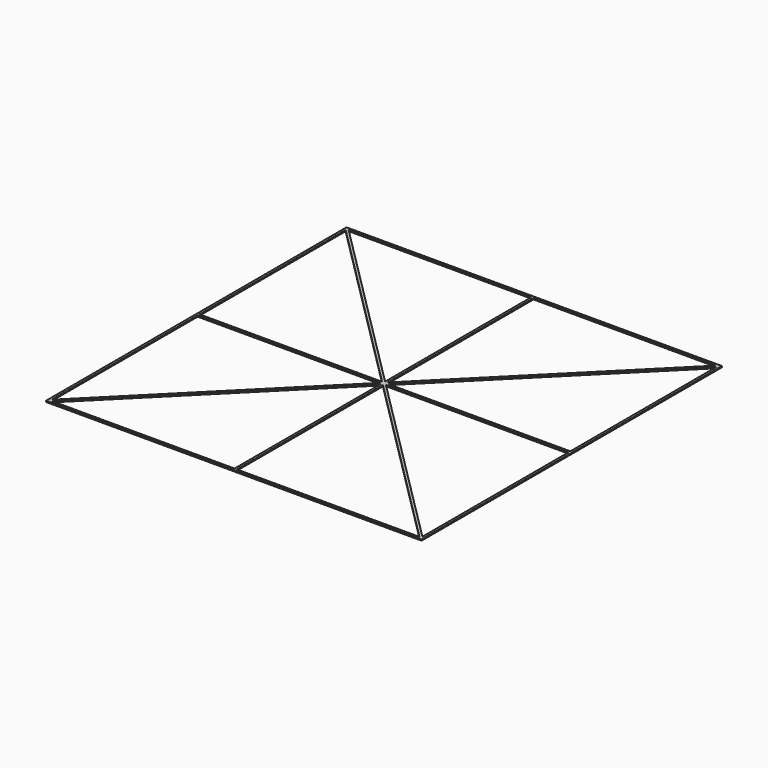
from build123d import *

# Parameters (mm, degrees)
F1_DEPTH = 0.5


# Not quite as in the source:
# - a pattern or mirror of a feature is missing from the dataset's text; its kind, count and spacing are read off the source's solid


with BuildPart() as f1:
    # F0 (on Top) → F1 (new body)
    with BuildSketch(Plane.XY):
        Polygon((160, 0), (0, 0), (0, -1), (0, -160), (160, -160), align=None)
        Polygon((1, -1.7071067812), (1, -1), (1.7071067812, -1), (79.5, -1), (80, -1), (80.5, -1), (158.2928932188, -1), (159, -1), (159, -1.7071067812), (159, -79.5), (159, -80.5), (159, -158.2928932188), (159, -159), (158.2928932188, -159), (80.5, -159), (80, -159), (79.5, -159), (1.7071067812, -159), (1, -159), (1, -158.2928932188), (1, -80.5), (1, -80), (1, -79.5), align=None, mode=Mode.SUBTRACT)
        Polygon((78.7928932188, -79.5), (1, -79.5), (1, -80), (1, -80.5), (78.7928932188, -80.5), (79.2928932188, -80), align=None)
        Polygon((159, -79.5), (81.2071067812, -79.5), (80.7071067812, -80), (81.2071067812, -80.5), (159, -80.5), align=None)
        Polygon((79.5, -78.7928932188), (1.7071067812, -1), (1.3535533906, -1.3535533906), (79.5, -79.5), align=None)
        Polygon((1.3535533906, -1.3535533906), (1, -1.7071067812), (78.7928932188, -79.5), (79.5, -79.5), align=None)
        Polygon((146.2407427602, -146.2407427602), (80.5, -80.5), (80.5, -81.2071067812), (145.8871893697, -146.5942961508), align=None)
        Polygon((81.2071067812, -80.5), (80.5, -80.5), (146.2407427602, -146.2407427602), (146.5942961508, -145.8871893697), align=None)
        Polygon((80, -1), (79.5, -1), (79.5, -78.7928932188), (80, -79.2928932188), align=None)
        Polygon((80.5, -1), (80, -1), (80, -79.2928932188), (80.5, -78.7928932188), align=None)
        Polygon((80, -80.7071067812), (79.5, -81.2071067812), (79.5, -159), (80, -159), align=None)
        Polygon((80.5, -81.2071067812), (80, -80.7071067812), (80, -159), (80.5, -159), align=None)
        Polygon((146.5942961508, -145.8871893697), (146.2407427602, -146.2407427602), (158.6464466094, -158.6464466094), (159, -158.2928932188), align=None)
        Polygon((158.6464466094, -158.6464466094), (146.2407427602, -146.2407427602), (145.8871893697, -146.5942961508), (158.2928932188, -159), align=None)
        Polygon((159, -1), (158.2928932188, -1), (149.7961722435, -9.4967209753), (150.1497256341, -9.8502743659), align=None)
        Polygon((159, -1.7071067812), (159, -1), (150.1497256341, -9.8502743659), (150.5032790247, -10.2038277565), align=None)
        Polygon((80, -79.2928932188), (79.5, -78.7928932188), (79.5, -79.5), (79.7928932188, -79.5), align=None)
        Polygon((79.5, -79.5), (78.7928932188, -79.5), (79.2928932188, -80), (79.5, -79.7928932188), align=None)
        Polygon((80.5, -78.7928932188), (80, -79.2928932188), (80.2071067812, -79.5), (80.5, -79.5), align=None)
        Polygon((79.5, -80.2071067812), (79.2928932188, -80), (78.7928932188, -80.5), (79.5, -80.5), align=None)
        Polygon((80, -80), (79.6464466094, -79.6464466094), (79.5, -79.7928932188), (79.5, -80.2071067812), (79.6464466094, -80.3535533906), align=None)
        Polygon((80.3535533906, -79.6464466094), (80, -80), (80.3535533906, -80.3535533906), (80.5, -80.2071067812), (80.5, -79.7928932188), align=None)
        Polygon((81.2071067812, -79.5), (80.5, -79.5), (80.5, -79.7928932188), (80.7071067812, -80), align=None)
        Polygon((79.7928932188, -80.5), (79.5, -80.5), (79.5, -81.2071067812), (80, -80.7071067812), align=None)
        Polygon((80.5, -80.5), (80.2071067812, -80.5), (80, -80.7071067812), (80.5, -81.2071067812), align=None)
        Polygon((80.7071067812, -80), (80.5, -80.2071067812), (80.5, -80.5), (81.2071067812, -80.5), align=None)
        Polygon((1.7071067812, -1), (1, -1), (1.3535533906, -1.3535533906), align=None)
        Polygon((1.3535533906, -1.3535533906), (1, -1), (1, -1.7071067812), align=None)
        Polygon((1.3535533906, -158.6464466094), (1, -158.2928932188), (1, -159), align=None)
        Polygon((1.3535533906, -158.6464466094), (1, -159), (1.7071067812, -159), align=None)
        Polygon((159, -158.2928932188), (158.6464466094, -158.6464466094), (159, -159), align=None)
        Polygon((159, -159), (158.6464466094, -158.6464466094), (158.2928932188, -159), align=None)
        Polygon((80, -79.5), (79.7928932188, -79.5), (79.6464466094, -79.6464466094), (80, -80), align=None)
        Polygon((80.2071067812, -79.5), (80, -79.5), (80, -80), (80.3535533906, -79.6464466094), align=None)
        Polygon((80.3535533906, -80.3535533906), (80, -80), (80, -80.5), (80.2071067812, -80.5), align=None)
        Polygon((80, -80.5), (80, -80), (79.6464466094, -80.3535533906), (79.7928932188, -80.5), align=None)
        Polygon((79.5, -79.7928932188), (79.2928932188, -80), (79.5, -80.2071067812), align=None)
        Polygon((80.7071067812, -80), (80.5, -79.7928932188), (80.5, -80.2071067812), align=None)
        Polygon((79.7928932188, -79.5), (79.5, -79.5), (79.6464466094, -79.6464466094), align=None)
        Polygon((79.6464466094, -79.6464466094), (79.5, -79.5), (79.5, -79.7928932188), align=None)
        Polygon((80.2071067812, -79.5), (80, -79.2928932188), (80, -79.5), align=None)
        Polygon((80, -79.5), (80, -79.2928932188), (79.7928932188, -79.5), align=None)
        Polygon((80.5, -79.5), (80.2071067812, -79.5), (80.3535533906, -79.6464466094), align=None)
        Polygon((79.6464466094, -80.3535533906), (79.5, -80.2071067812), (79.5, -80.5), align=None)
        Polygon((80.5, -79.7928932188), (80.5, -79.5), (80.3535533906, -79.6464466094), align=None)
        Polygon((79.6464466094, -80.3535533906), (79.5, -80.5), (79.7928932188, -80.5), align=None)
        Polygon((80, -80.7071067812), (80, -80.5), (79.7928932188, -80.5), align=None)
        Polygon((80.2071067812, -80.5), (80, -80.5), (80, -80.7071067812), align=None)
        Polygon((80.5, -80.5), (80.3535533906, -80.3535533906), (80.2071067812, -80.5), align=None)
        Polygon((80.5, -80.2071067812), (80.3535533906, -80.3535533906), (80.5, -80.5), align=None)
    extrude(amount=F1_DEPTH)

    # F1_copies: F1 across plane


with BuildPart() as f1_1:
    add(f1.part)
    add(f1.part.mirror(Plane(origin=(80, 0, 0), x_dir=(0, 0, 1), z_dir=(1, 0, 0))))


solid = f1_1.part
